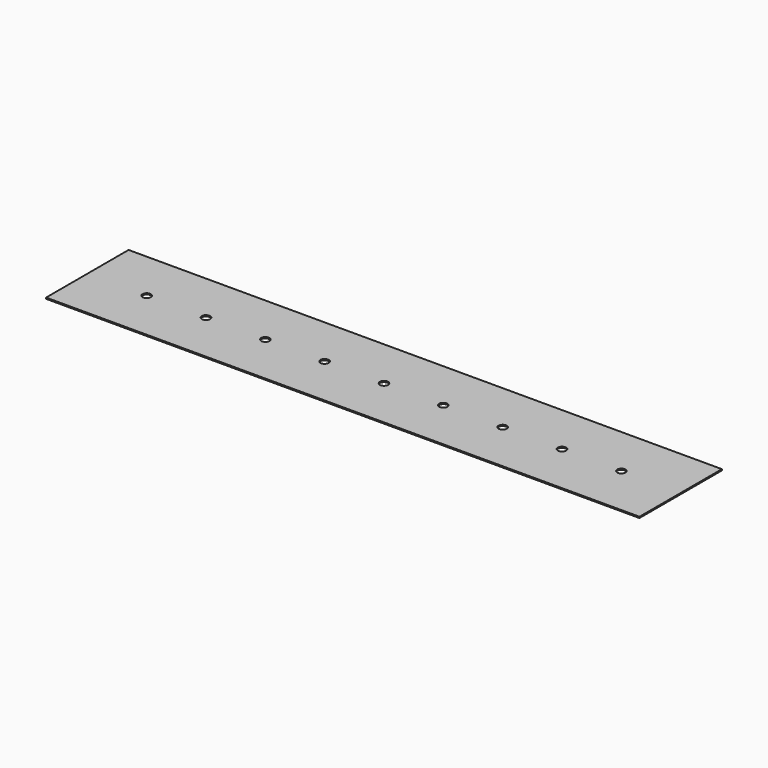
from build123d import *

# Parameters (mm, degrees)
F0_W     = 250
F0_H     = 43.4334799647
F0_R     = 1.75
F2_DEPTH = 0.5


# Not quite as in the source:
# - the program builds the solid bodies; features that only make, move or delete a surface that nothing else refers to are left out


with BuildPart() as f2:
    # F0 (on Top) → F2 (new body)
    with BuildSketch(Plane.XY):
        with Locations((-14.8854096483, -21.7167399824)):
            Rectangle(F0_W, F0_H)
        with Locations((-114.8854096483, -21.7167399824)):
            Circle(F0_R, mode=Mode.SUBTRACT)
        with Locations((-89.8854096483, -21.7167399824)):
            Circle(F0_R, mode=Mode.SUBTRACT)
        with Locations((-64.8854096483, -21.7167399824)):
            Circle(F0_R, mode=Mode.SUBTRACT)
        with Locations((-39.8854096483, -21.7167399824)):
            Circle(F0_R, mode=Mode.SUBTRACT)
        with Locations((-14.8854096483, -21.7167399824)):
            Circle(F0_R, mode=Mode.SUBTRACT)
        with Locations((10.1145903517, -21.7167399824)):
            Circle(F0_R, mode=Mode.SUBTRACT)
        with Locations((35.1145903517, -21.7167399824)):
            Circle(F0_R, mode=Mode.SUBTRACT)
        with Locations((60.1145903517, -21.7167399824)):
            Circle(F0_R, mode=Mode.SUBTRACT)
        with Locations((85.1145903517, -21.7167399824)):
            Circle(F0_R, mode=Mode.SUBTRACT)
    extrude(amount=F2_DEPTH)


solid = f2.part
